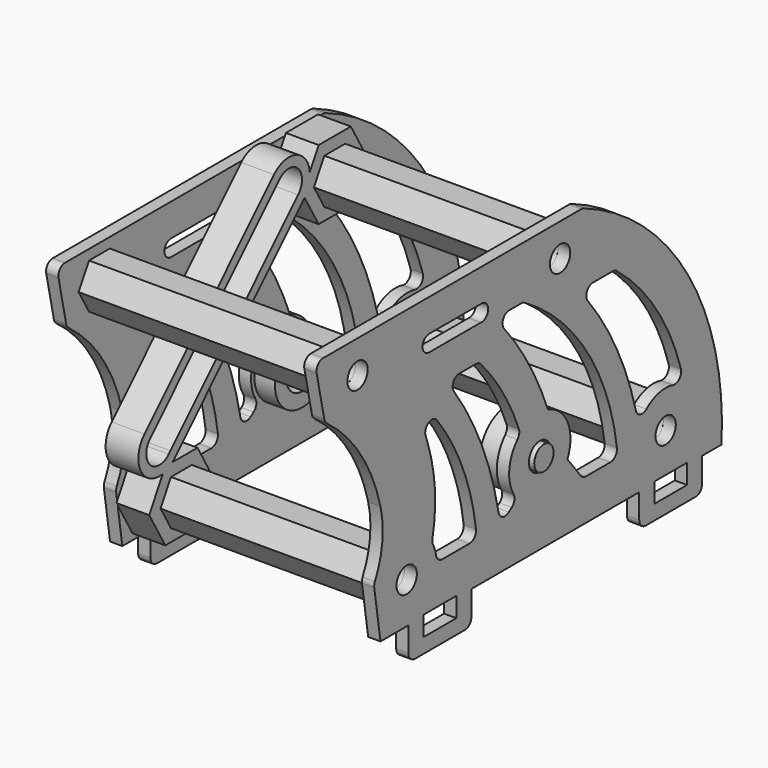
from build123d import *

# Parameters (mm, degrees)
F0_R      = 1.55
F0_W      = 5
F0_H      = 2.4
F0_R_2    = 1.675
F1_DEPTH  = 1.5
F2_R      = 1
F3_R      = 1.55
F4_DEPTH  = 30
F5_R      = 1.475
F6_DEPTH  = 2
F5_R_2    = 4.175
F5_R_3    = 1.675
F7_DEPTH  = 2.5
F8_R      = 2.45
F9_DEPTH  = 1
F10_R     = 0.8
F14_DEPTH = 4


# Not quite as in the source:
# - a feature names something its author has since deleted; it is built from what else it names


with BuildPart() as f1:
    # F0 (on Right) → F1 (new body)
    with BuildSketch(Plane.YZ):
        with BuildLine():
            Line((22.1878419101, 14), (25.1370414712, 14))
            ThreePointArc((25.1370414712, 14), (19.9791691176, 34.395640327), (3.9321385681, 48))
            Line((3.9321385681, 48), (-36.8864646358, 48))
            Line((-36.8864646358, 48), (-35.3864646358, 41))
            ThreePointArc((-35.3864646358, 41), (-30.0291716069, 35.5029592597), (-26.8864646358, 28.5))
            ThreePointArc((-26.8864646358, 28.5), (-26.6271187765, 24.4050817676), (-27.8864646358, 20.5))
            Line((-27.8864646358, 20.5), (-26.8864646358, 14))
            Line((-26.8864646358, 14), (-22.6117424995, 14))
            Line((-22.6117424995, 14), (-22.6117424995, 11))
            ThreePointArc((-22.6117424995, 11), (-22.3188492807, 10.2928932188), (-21.6117424995, 10))
            Line((-21.6117424995, 10), (-14.0117424995, 10))
            ThreePointArc((-14.0117424995, 10), (-13.3046357183, 10.2928932188), (-13.0117424995, 11))
            Line((-13.0117424995, 11), (-13.0117424995, 14))
            Line((-13.0117424995, 14), (12.5878419101, 14))
            Line((12.5878419101, 14), (12.5878419101, 11))
            ThreePointArc((12.5878419101, 11), (12.8807351289, 10.2928932188), (13.5878419101, 10))
            Line((13.5878419101, 10), (21.1878419101, 10))
            ThreePointArc((21.1878419101, 10), (21.8949486913, 10.2928932188), (22.1878419101, 11))
            Line((22.1878419101, 11), (22.1878419101, 14))
        make_face()
        with Locations((-22.8864646358, 19)):
            Circle(F0_R, mode=Mode.SUBTRACT)
        with Locations((-17.8117424995, 13)):
            Rectangle(F0_W, F0_H, mode=Mode.SUBTRACT)
        with BuildLine():
            Line((-12.184658767, 19), (-18.3364646358, 19))
            ThreePointArc((-18.3364646358, 19), (-18.5166935868, 20.267912055), (-19.0431024289, 21.4353781938))
            ThreePointArc((-19.0431024289, 21.4353781938), (-18.5431011345, 25.9570172572), (-19.1322689351, 30.4679043559))
            ThreePointArc((-19.1322689351, 30.4679043559), (-20.5616008853, 34.7479451576), (-22.6167159041, 38.7651881608))
            ThreePointArc((-22.6167159041, 38.7651881608), (-15.4555559224, 29.9092335374), (-12.184658767, 19))
        make_face(mode=Mode.SUBTRACT)
        with BuildLine():
            Line((-6.0378868771, 20.8520555699), (-8.6154459624, 19))
            ThreePointArc((-8.6154459624, 19), (-11.5114554094, 28.9926085981), (-16.8864646358, 37.9003789774))
            Line((-16.8864646358, 37.9003789774), (-11.8864646358, 37.9003789774))
            ThreePointArc((-11.8864646358, 37.9003789774), (-8.1809613239, 33.0887444148), (-5.5397744404, 27.6200412955))
            ThreePointArc((-5.5397744404, 27.6200412955), (-7.2439676654, 24.3431440842), (-6.0378868771, 20.8520555699))
        make_face(mode=Mode.SUBTRACT)
        with Locations((17.3878419101, 13)):
            Rectangle(F0_W, F0_H, mode=Mode.SUBTRACT)
        with Locations((16.6135353642, 19)):
            Circle(F0_R, mode=Mode.SUBTRACT)
        with Locations((-2.5815780273, 24)):
            Circle(F0_R_2, mode=Mode.SUBTRACT)
        with Locations((-30.3864646358, 44)):
            Circle(F0_R, mode=Mode.SUBTRACT)
        with BuildLine():
            ThreePointArc((-11.4631414181, 44.037760675), (-10.4615955247, 42.9789551855), (-11.5743920625, 42.037760675))
            Line((-11.5743920625, 42.037760675), (-19.5743920625, 42.037760675))
            ThreePointArc((-19.5743920625, 42.037760675), (-20.4646873114, 43.0903778115), (-19.4631414181, 44.037760675))
            Line((-19.4631414181, 44.037760675), (-11.4631414181, 44.037760675))
        make_face(mode=Mode.SUBTRACT)
        with BuildLine():
            ThreePointArc((-5.1485669028, 41.6), (4.8029226996, 32.0404916878), (9.315341233, 19))
            Line((9.315341233, 19), (3.9649060927, 19))
            Line((3.9649060927, 19), (1.6351427929, 21.9813641922))
            ThreePointArc((1.6351427929, 21.9813641922), (1.6734803304, 25.9365183635), (-1.3340420549, 28.505472117))
            ThreePointArc((-1.3340420549, 28.505472117), (-4.7728105503, 35.4493931323), (-9.4858990272, 41.6))
            Line((-9.4858990272, 41.6), (-5.1485669028, 41.6))
        make_face(mode=Mode.SUBTRACT)
        with BuildLine():
            ThreePointArc((8.8754455206, 39.3779618357), (15.6611772839, 31.8700604828), (19.5087734612, 22.5099994817))
            ThreePointArc((19.5087734612, 22.5099994817), (15.6517553527, 23.4471877866), (12.5266661468, 21))
            ThreePointArc((12.5266661468, 21), (9.150215671, 30.7860969819), (3.3754455206, 39.3779618357))
            Line((3.3754455206, 39.3779618357), (8.8754455206, 39.3779618357))
        make_face(mode=Mode.SUBTRACT)
        with Locations((0.5111069477, 44)):
            Circle(F0_R, mode=Mode.SUBTRACT)
    extrude(amount=F1_DEPTH)

    # F2
    f2_edges = [f1.edges().sort_by_distance(p)[0] for p in [
        (0.75, -36.886465, 48),
        (0.75, -35.386465, 41),
        (0.75, -27.886465, 20.5),
        (0.75, 3.932139, 48),
        (0.75, -12.184659, 19),
        (0.75, -18.336465, 19),
        (0.75, -8.615446, 19),
        (0.75, -9.485899, 41.6),
        (0.75, -5.148567, 41.6),
        (0.75, 19.508773, 22.509999),
        (0.75, 12.526666, 21),
        (0.75, 9.315341, 19),
        (0.75, -22.616716, 38.765188),
        (0.75, -19.043102, 21.435378),
        (0.75, -16.886465, 37.900379),
        (0.75, -11.886465, 37.900379),
        (0.75, -5.539774, 27.620041),
        (0.75, -6.037887, 20.852056),
        (0.75, 3.964906, 19),
        (0.75, 3.375446, 39.377962),
        (0.75, 8.875446, 39.377962),
    ]]
    fillet(f2_edges, radius=F2_R)


with BuildPart() as f4:
    # F3 (on face) → F4 (new body)
    with BuildSketch(Plane(origin=(0, 0, 0), x_dir=(0, -1, 0), z_dir=(-1, 0, 0))):
        Polygon((-15.0258221239, 21.75), (-18.2012486045, 21.75), (-19.7889618447, 19), (-18.2012486045, 16.25), (-15.0258221239, 16.25), (-13.4381088836, 19), align=None)
        with Locations((-16.6135353642, 19)):
            Circle(F3_R, mode=Mode.SUBTRACT)
    extrude(amount=F4_DEPTH)


with BuildPart() as f4b:
    # F3 (on face) → F4, piece 2 (new body)
    with BuildSketch(Plane(origin=(0, 0, 0), x_dir=(0, -1, 0), z_dir=(-1, 0, 0))):
        Polygon((24.4741778761, 21.75), (21.2987513955, 21.75), (19.7110381553, 19), (21.2987513955, 16.25), (24.4741778761, 16.25), (26.0618911164, 19), align=None)
        with Locations((22.8864646358, 19)):
            Circle(F3_R, mode=Mode.SUBTRACT)
    extrude(amount=F4_DEPTH)


with BuildPart() as f4c:
    # F3 (on face) → F4, piece 3 (new body)
    with BuildSketch(Plane(origin=(0, 0, 0), x_dir=(0, -1, 0), z_dir=(-1, 0, 0))):
        Polygon((1.0766062926, 46.75), (-2.098820188, 46.75), (-3.6865334282, 44), (-2.098820188, 41.25), (1.0766062926, 41.25), (2.6643195329, 44), align=None)
        with Locations((-0.5111069477, 44)):
            Circle(F3_R, mode=Mode.SUBTRACT)
    extrude(amount=F4_DEPTH)


with BuildPart() as f4d:
    # F3 (on face) → F4, piece 4 (new body)
    with BuildSketch(Plane(origin=(0, 0, 0), x_dir=(0, -1, 0), z_dir=(-1, 0, 0))):
        Polygon((33.5618911164, 44), (31.9741778761, 46.75), (28.7987513955, 46.75), (27.2110381553, 44), (28.7987513955, 41.25), (31.9741778761, 41.25), align=None)
        with Locations((30.3864646358, 44)):
            Circle(F3_R, mode=Mode.SUBTRACT)
    extrude(amount=F4_DEPTH)


with BuildPart() as f6:
    # F5 (on face) → F6 (new body)
    with BuildSketch(Plane(origin=(0, 0, 0), x_dir=(0, -1, 0), z_dir=(-1, 0, 0))):
        with Locations((2.5815780273, 24)):
            Circle(F5_R)
    extrude(amount=-F6_DEPTH)

    # F5 (on face) → F7 (join)
    with BuildSketch(Plane(origin=(0, 0, 0), x_dir=(0, -1, 0), z_dir=(-1, 0, 0))):
        with Locations((2.5815780273, 24)):
            Circle(F5_R_2)
        with Locations((2.5815780273, 24)):
            Circle(F5_R_3, mode=Mode.SUBTRACT)
        with Locations((2.5815780273, 24)):
            Circle(F5_R_3)
        with Locations((2.5815780273, 24)):
            Circle(F5_R, mode=Mode.SUBTRACT)
        with Locations((2.5815780273, 24)):
            Circle(F5_R)
    extrude(amount=F7_DEPTH)

    # F8 (on face) → F9 (cut)
    with BuildSketch(Plane(origin=(-2.5, 0, 0), x_dir=(0, -1, 0), z_dir=(-1, 0, 0))):
        with Locations((2.5815780273, 24)):
            Circle(F8_R)
    extrude(amount=-F9_DEPTH, mode=Mode.SUBTRACT)

    # F10
    f10_edges = [f6.edges().sort_by_distance(p)[0] for p in [
        (-1.5, -0.131578, 24),
        (0, -1.106578, 24),
    ]]
    fillet(f10_edges, radius=F10_R)


with BuildPart() as f12_1:
    # F12: instance of F1
    add(f1.part.mirror(Plane(origin=(-15, -30.3864646358, 44), x_dir=(0, 1, 0), z_dir=(1, 0, 0))))


with BuildPart() as f12_2:
    # F12: instance of F6
    add(f6.part.mirror(Plane(origin=(-15, -30.3864646358, 44), x_dir=(0, 1, 0), z_dir=(1, 0, 0))))


with BuildPart() as f14:
    # F13 (on face) → F14 (new body)
    with BuildSketch(Plane(origin=(-30, 0, 0), x_dir=(0, -1, 0), z_dir=(-1, 0, 0))):
        with BuildLine():
            Line((1.9426316964, 48.25), (-2.9648455917, 48.25))
            Line((-2.9648455917, 48.25), (-5.4185842358, 44))
            Line((-5.4185842358, 44), (-2.9648455917, 39.75))
            Line((-2.9648455917, 39.75), (1.9426316964, 39.75))
            Line((1.9426316964, 39.75), (4.0895659873, 43.4685992723))
            ThreePointArc((4.0895659873, 43.4685992723), (3.4435761842, 44.6000551469), (3.3021549231, 45.8952366973))
            Line((3.3021549231, 45.8952366973), (1.9426316964, 48.25))
        make_face()
        Polygon((-2.098820188, 46.75), (1.0766062926, 46.75), (2.6643195329, 44), (1.0766062926, 41.25), (-2.098820188, 41.25), (-3.6865334282, 44), align=None, mode=Mode.SUBTRACT)
        with BuildLine():
            Line((4.3963703404, 44), (3.3021549231, 45.8952366973))
            ThreePointArc((3.3021549231, 45.8952366973), (3.4435761842, 44.6000551469), (4.0895659873, 43.4685992723))
            Line((4.0895659873, 43.4685992723), (4.3963703404, 44))
        make_face()
        with BuildLine():
            ThreePointArc((8.7550268128, 47.8455068877), (5.4096879828, 48.6007977414), (3.3021549231, 45.8952366973))
            Line((3.3021549231, 45.8952366973), (4.3963703404, 44))
            Line((4.3963703404, 44), (4.0895659873, 43.4685992723))
            ThreePointArc((4.0895659873, 43.4685992723), (4.1535836874, 43.3982964794), (4.2196618313, 43.3299266941))
            Line((4.2196618313, 43.3299266941), (23.9753251782, 23.4877049))
            ThreePointArc((23.9753251782, 23.4877049), (24.1042995608, 23.3651740881), (24.2398839281, 23.25))
            Line((24.2398839281, 23.25), (25.3402032799, 23.25))
            Line((25.3402032799, 23.25), (25.7223285765, 22.5881395713))
            ThreePointArc((25.7223285765, 22.5881395713), (29.0879954501, 24.2805565938), (28.5106901597, 28.0032850936))
            Line((28.5106901597, 28.0032850936), (8.7550268128, 47.8455068877))
        make_face()
        with BuildLine():
            Line((24.8257061122, 24.3343761863), (24.5601446323, 24.6011012106))
            Line((24.5601446323, 24.6011012106), (5.0700427653, 44.1765979804))
            ThreePointArc((5.0700427653, 44.1765979804), (5.0762255115, 47.0050183476), (7.9046458787, 46.9988356014))
            Line((7.9046458787, 46.9988356014), (27.6603092256, 27.1566138073))
            ThreePointArc((27.6603092256, 27.1566138073), (27.6541264794, 24.3281934401), (24.8257061122, 24.3343761863))
        make_face(mode=Mode.SUBTRACT)
        with BuildLine():
            Line((27.7939419239, 19), (25.7223285765, 22.5881395713))
            ThreePointArc((25.7223285765, 22.5881395713), (24.938434945, 22.8234939687), (24.2398839281, 23.25))
            Line((24.2398839281, 23.25), (20.4327259918, 23.25))
            Line((20.4327259918, 23.25), (17.9789873477, 19))
            Line((17.9789873477, 19), (20.4327259918, 14.75))
            Line((20.4327259918, 14.75), (25.3402032799, 14.75))
            Line((25.3402032799, 14.75), (27.7939419239, 19))
        make_face()
        Polygon((21.2987513955, 21.75), (24.4741778761, 21.75), (26.0618911164, 19), (24.4741778761, 16.25), (21.2987513955, 16.25), (19.7110381553, 19), align=None, mode=Mode.SUBTRACT)
        with BuildLine():
            ThreePointArc((24.2398839281, 23.25), (24.938434945, 22.8234939687), (25.7223285765, 22.5881395713))
            Line((25.7223285765, 22.5881395713), (25.3402032799, 23.25))
            Line((25.3402032799, 23.25), (24.2398839281, 23.25))
        make_face()
    extrude(amount=-F14_DEPTH)


solid = Compound([f1.part, f4.part, f4b.part, f4c.part, f4d.part, f6.part, f12_1.part, f12_2.part, f14.part])
